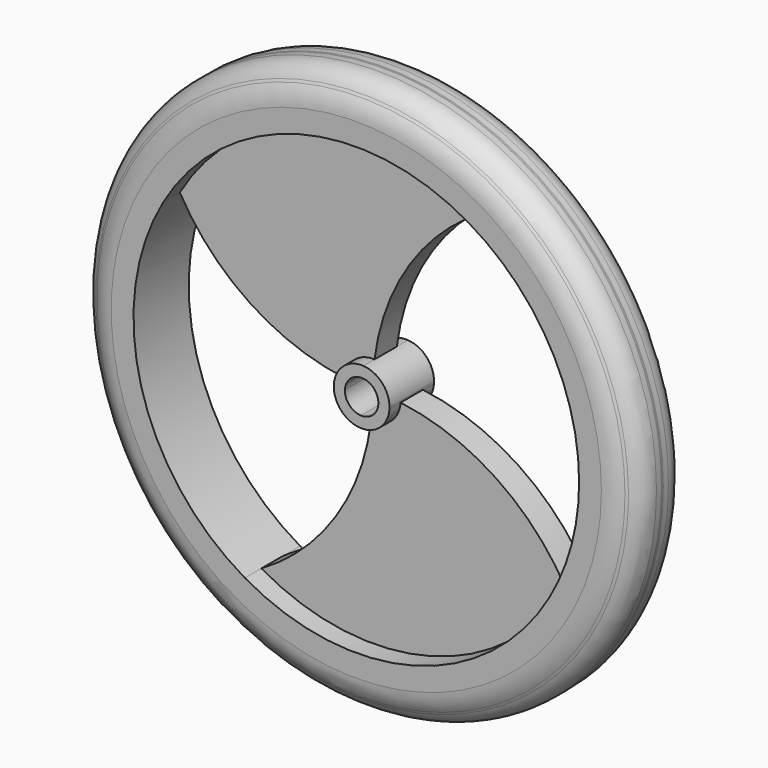
from build123d import *

# Parameters (mm, degrees)
F0_R     = 63.5
F1_DEPTH = 7.874
F2_DEPTH = 3.175
F4_R     = 7.62
F5_DEPTH = 6.35
F7_R     = 5.08


# Not quite as in the source:
# - a fillet or chamfer that OpenCascade refuses, or shapes differently, is made with other operations: its cross-section is extruded or revolved along the edge and cut away or added
# - the program builds the solid bodies; features that only make, move or delete a surface that nothing else refers to are left out


with BuildPart() as f1:
    # F0 (on Front) → F1 (new body, symmetric)
    with BuildSketch(Plane.XZ):
        Circle(F0_R)
        with BuildLine():
            ThreePointArc((25.4, 43.994091), (43.994091, 25.4), (50.8, 0))
            ThreePointArc((50.8, 0), (49.069032, -13.148007), (43.994091, -25.4))
            ThreePointArc((43.994091, -25.4), (13.148007, -49.069032), (-25.4, -43.994091))
            ThreePointArc((-25.4, -43.994091), (-49.069032, -13.148007), (-43.994091, 25.4))
            ThreePointArc((-43.994091, 25.4), (-13.148007, 49.069032), (25.4, 43.994091))
        make_face(mode=Mode.SUBTRACT)
    extrude(amount=F1_DEPTH, both=True)

    # F0 (on Front) → F2 (join, symmetric)
    with BuildSketch(Plane.XZ):
        with BuildLine():
            ThreePointArc((-25.4, -43.994091), (13.148007, -49.069032), (43.994091, -25.4))
            ThreePointArc((43.994091, -25.4), (28.099973, -8.47942), (6.337586, -0.396875))
            ThreePointArc((6.337586, -0.396875), (4.200717, -4.761983), (-0.396875, -6.337586))
            ThreePointArc((-0.396875, -6.337586), (-8.47942, -28.099973), (-25.4, -43.994091))
        make_face()
        with BuildLine():
            ThreePointArc((0.396875, 6.337586), (8.47942, 28.099973), (25.4, 43.994091))
            ThreePointArc((25.4, 43.994091), (-13.148007, 49.069032), (-43.994091, 25.4))
            ThreePointArc((-43.994091, 25.4), (-28.099973, 8.47942), (-6.337586, 0.396875))
            ThreePointArc((-6.337586, 0.396875), (-4.200717, 4.761983), (0.396875, 6.337586))
        make_face()
    extrude(amount=F2_DEPTH, both=True)

    # F4
    f4_edges = [f1.edges().sort_by_distance(p)[0] for p in [
        (-63.5, 7.874, 0),
        (-63.5, -7.874, 0),
    ]]
    fillet(f4_edges, radius=F4_R)

    # F0 (on Front) → F5 (join, symmetric)
    with BuildSketch(Plane.XZ):
        Circle(F0_R)
        with BuildLine():
            ThreePointArc((25.4, 43.994091), (43.994091, 25.4), (50.8, 0))
            ThreePointArc((50.8, 0), (49.069032, -13.148007), (43.994091, -25.4))
            ThreePointArc((43.994091, -25.4), (13.148007, -49.069032), (-25.4, -43.994091))
            ThreePointArc((-25.4, -43.994091), (-49.069032, -13.148007), (-43.994091, 25.4))
            ThreePointArc((-43.994091, 25.4), (-13.148007, 49.069032), (25.4, 43.994091))
        make_face(mode=Mode.SUBTRACT)
        with BuildLine():
            ThreePointArc((6.35, 0), (4.628318, 4.347548), (0.396875, 6.337586))
            ThreePointArc((0.396875, 6.337586), (0.25404, 5.074042), (0.142875, 3.80732))
            ThreePointArc((0.142875, 3.80732), (2.744126, 2.64308), (3.81, 0))
            ThreePointArc((3.81, 0), (3.80933, -0.07145), (3.80732, -0.142875))
            ThreePointArc((3.80732, -0.142875), (5.074042, -0.25404), (6.337586, -0.396875))
            ThreePointArc((6.337586, -0.396875), (6.346896, -0.198535), (6.35, 0))
        make_face()
        with BuildLine():
            ThreePointArc((0.142875, 3.80732), (0.25404, 5.074042), (0.396875, 6.337586))
            ThreePointArc((0.396875, 6.337586), (-4.200717, 4.761983), (-6.337586, 0.396875))
            ThreePointArc((-6.337586, 0.396875), (-5.074042, 0.25404), (-3.80732, 0.142875))
            ThreePointArc((-3.80732, 0.142875), (-2.591154, 2.79321), (0.142875, 3.80732))
        make_face()
        with BuildLine():
            ThreePointArc((-3.80732, 0.142875), (-5.074042, 0.25404), (-6.337586, 0.396875))
            ThreePointArc((-6.337586, 0.396875), (-4.761983, -4.200717), (-0.396875, -6.337586))
            ThreePointArc((-0.396875, -6.337586), (-0.25404, -5.074042), (-0.142875, -3.80732))
            ThreePointArc((-0.142875, -3.80732), (-2.79321, -2.591154), (-3.80732, 0.142875))
        make_face()
        with BuildLine():
            ThreePointArc((-0.396875, -6.337586), (4.200717, -4.761983), (6.337586, -0.396875))
            ThreePointArc((6.337586, -0.396875), (5.074042, -0.25404), (3.80732, -0.142875))
            ThreePointArc((3.80732, -0.142875), (2.591154, -2.79321), (-0.142875, -3.80732))
            ThreePointArc((-0.142875, -3.80732), (-0.25404, -5.074042), (-0.396875, -6.337586))
        make_face()
    extrude(amount=F5_DEPTH, both=True)

    # F6: fillet of radius 5.08 on 2 edges, made by hand

    # F6_s1 → F6_t2 (revolve, cut)
    with BuildSketch(Plane.XY):
        with BuildLine():
            ThreePointArc((63.5, 1.694103), (62.670233, 4.476534), (60.452, 6.35))
            Line((60.452, 6.35), (60.49264, 6.443118))
            ThreePointArc((60.49264, 6.443118), (61.976, 6.4516), (63.5, 6.4516))
            Line((63.5, 6.4516), (63.6016, 6.35))
            Line((63.6016, 6.35), (63.6016, 1.694103))
            Line((63.6016, 1.694103), (63.5, 1.694103))
        make_face()
    revolve(axis=Axis((0, 6.35, 0), (0, -1, 0)), mode=Mode.SUBTRACT)

    # F6_s3 → F6_t4 (revolve, cut)
    with BuildSketch(Plane.XY):
        with BuildLine():
            ThreePointArc((63.5, -1.694103), (62.670233, -4.476534), (60.452, -6.35))
            Line((60.452, -6.35), (60.49264, -6.443118))
            ThreePointArc((60.49264, -6.443118), (61.976, -6.4516), (63.5, -6.4516))
            Line((63.5, -6.4516), (63.6016, -6.35))
            Line((63.6016, -6.35), (63.6016, -1.694103))
            Line((63.6016, -1.694103), (63.5, -1.694103))
        make_face()
    revolve(axis=Axis((0, -6.35, 0), (0, -1, 0)), mode=Mode.SUBTRACT)

    # F7
    f7_edges = [f1.edges().sort_by_distance(p)[0] for p in [
        (-60.452, -6.35, 0),
        (-60.452, 6.35, 0),
    ]]
    fillet(f7_edges, radius=F7_R)


solid = f1.part
